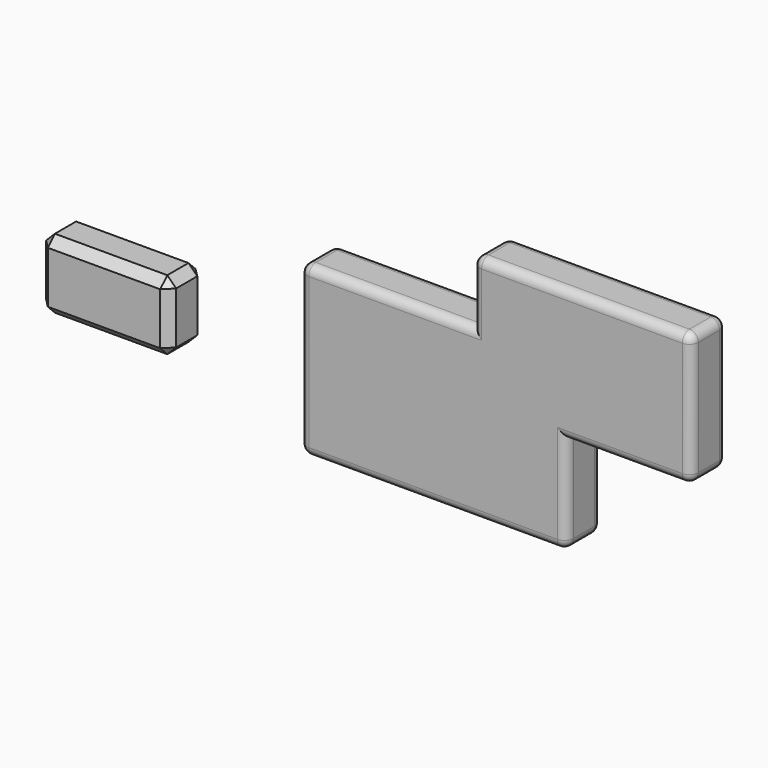
from build123d import *

# Parameters (mm, degrees)
F0_W     = 74.8927108943
F0_H     = 40.061917156
F1_DEPTH = 25.4
F0_W_2   = 83.2777917385
F0_H_2   = 54.8879876733
F0_W_3   = 53.8076832891
F0_H_3   = 40.1005172171
F2_R     = 5.08
F3_R     = 5.08
F4_R     = 5.08
F5_R     = 5.08
F6_R     = 5.08
F7_R     = 5.08
F9_R     = 5.08
F10_R    = 5.08
F12_SIZE = 5.08


# Not quite as in the source:
# - a feature of the source that left no trace in its solid (it failed there, or was rolled back) is left out


with BuildPart() as f1:
    # F0 (on Front) → F1 (new body)
    with BuildSketch(Plane.XZ):
        with Locations((-88.5540191084, -20.030958578)):
            Rectangle(F0_W, F0_H)
    extrude(amount=F1_DEPTH)

    # F12
    f12_edges = [f1.edges().sort_by_distance(p)[0] for p in [
        (-51.107664, -12.7, 0),
        (-126.000375, -12.7, 0),
        (-88.554019, 0, 0),
        (-88.554019, -25.4, 0),
        (-51.107664, -12.7, -40.061917),
        (-51.107664, 0, -20.030959),
        (-51.107664, -25.4, -20.030959),
        (-126.000375, 0, -20.030959),
        (-88.554019, 0, -40.061917),
        (-126.000375, -12.7, -40.061917),
        (-88.554019, -25.4, -40.061917),
        (-126.000375, -25.4, -20.030959),
    ]]
    chamfer(f12_edges, length=F12_SIZE)


with BuildPart() as f1b:
    # F0 (on Front) → F1, piece 2 (new body)
    with BuildSketch(Plane.XZ):
        with Locations((-227.9445976019, -110.2393232286)):
            Rectangle(F0_W_2, F0_H_2)
    extrude(amount=F1_DEPTH)


with BuildPart() as f1c:
    # F0 (on Front) → F1, piece 3 (new body)
    with BuildSketch(Plane.XZ):
        Polygon((249.6970742941, -5.7757184841), (249.6970742941, 70.4710111022), (123.860694468, 70.4710111022), (123.860694468, 34.324798733), (177.6683777571, 34.324798733), (177.6683777571, -5.7757184841), align=None)
        with Locations((150.7645361125, 14.2745401245)):
            Rectangle(F0_W_3, F0_H_3)
        Polygon((123.860694468, -5.7757184841), (123.860694468, 34.324798733), (24.3443846703, 34.324798733), (24.3443846703, -62.544003129), (177.6683777571, -62.544003129), (177.6683777571, -5.7757184841), align=None)
    extrude(amount=F1_DEPTH)

    # F2
    f2_edges = [f1c.edges().sort_by_distance(p)[0] for p in [
        (249.697074, 0, 32.347646),
    ]]
    fillet(f2_edges, radius=F2_R)

    # F3
    f3_edges = [f1c.edges().sort_by_distance(p)[0] for p in [
        (211.142726, 0, -5.775718),
    ]]
    fillet(f3_edges, radius=F3_R)

    # F4
    f4_edges = [f1c.edges().sort_by_distance(p)[0] for p in [
        (177.668378, 0, -34.159861),
    ]]
    fillet(f4_edges, radius=F4_R)

    # F5
    f5_edges = [f1c.edges().sort_by_distance(p)[0] for p in [
        (98.466381, 0, -62.544003),
    ]]
    fillet(f5_edges, radius=F5_R)

    # F6
    f6_edges = [f1c.edges().sort_by_distance(p)[0] for p in [
        (24.344385, 0, -11.569602),
    ]]
    fillet(f6_edges, radius=F6_R)

    # F7
    f7_edges = [f1c.edges().sort_by_distance(p)[0] for p in [
        (76.64254, 0, 34.324799),
    ]]
    fillet(f7_edges, radius=F7_R)

    # F9
    f9_edges = [f1c.edges().sort_by_distance(p)[0] for p in [
        (123.860694, 0, 31.784799),
    ]]
    fillet(f9_edges, radius=F9_R)

    # F10
    f10_edges = [f1c.edges().sort_by_distance(p)[0] for p in [
        (24.344385, -25.4, -14.109602),
        (25.832282, -25.4, 32.836901),
        (25.832282, -25.4, -61.056106),
        (76.64254, -25.4, 34.324799),
        (101.006381, -25.4, -62.544003),
        (123.860694, -25.4, 52.397905),
        (176.18048, -25.4, -61.056106),
        (186.778884, -25.4, 70.471011),
        (177.668378, -25.4, -31.619861),
        (249.697074, -25.4, 34.887646),
        (211.142726, -25.4, -5.775718),
        (248.209177, -25.4, -4.287821),
        (186.778884, 0, 70.471011),
        (125.348592, -1.487898, 70.471011),
        (248.209177, -1.487898, 70.471011),
    ]]
    fillet(f10_edges, radius=F10_R)


solid = Compound([f1.part, f1c.part])
